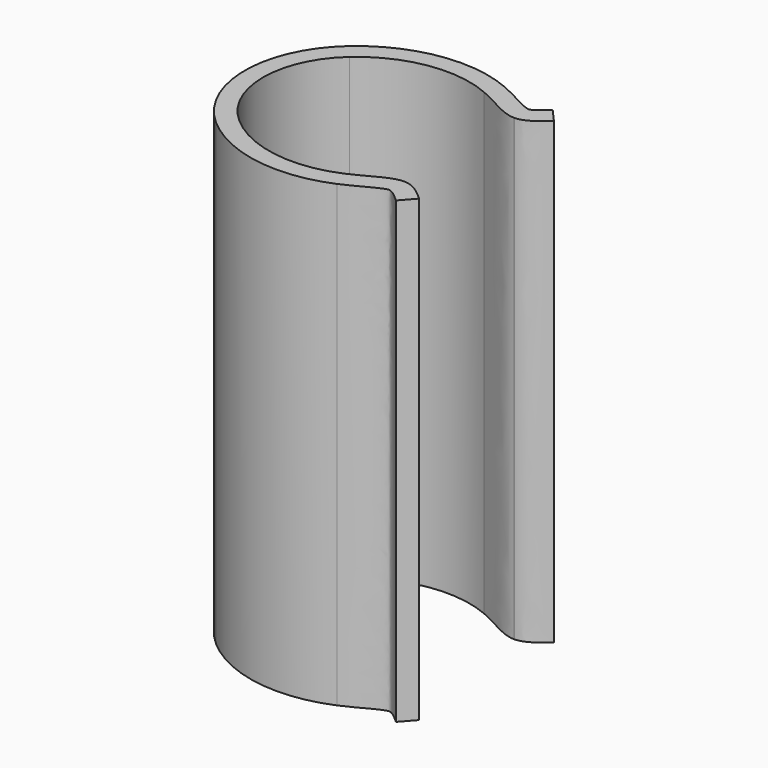
from build123d import *

# Parameters (mm, degrees)
F1_DEPTH = 50


# Not quite as in the source:
# - the dataset's text gives a spline's control points without its knots; the knots are read off the source's solid


with BuildPart() as f1:
    # F0 (on Top) → F1 (new body)
    with BuildSketch(Plane.XY):
        with BuildLine():
            ThreePointArc((13.0144933843, -2.085252316), (6.205255597, -2.9274153897), (0, 0))
            ThreePointArc((0, 0), (-3.3856217223, 7.5), (0, 15))
            ThreePointArc((0, 15), (6.205255597, 17.9274153897), (13.0144933843, 17.085252316))
            add(Edge.make_bspline(
                [(13.0144933843, 17.085252316), (14.9188937147, 16.2688716797), (16.5381459826, 15.0282447438), (17.9057964085, 15)],
                knots=[0, 0, 0, 0, 0.5457987429, 0.5457987429, 0.5457987429, 0.5457987429], degree=3))
            Line((17.9057964085, 15), (18, 15))
            add(Edge.make_bspline(
                [(18, 15), (19.0972191031, 15.0230880512), (20.0302273141, 15.8645970051), (20.9385249764, 16.6705846786)],
                knots=[0.5583835876, 0.5583835876, 0.5583835876, 0.5583835876, 1, 1, 1, 1], degree=3))
            Line((20.9385249764, 16.6705846786), (19.6110748236, 18.1665379172))
            add(Edge.make_bspline(
                [(13.8027239443, 18.9233743561), (14.3068240335, 18.7072663795), (15.238145762, 18.2426302327), (16.2240017083, 17.7036956521), (16.8916980315, 17.3645051566), (17.3205970551, 17.1709950677), (17.6036754274, 17.0697214684), (17.7738298239, 17.0243049098), (17.8699589675, 17.0058001031), (17.9347425496, 16.9993397818), (17.9615712094, 16.9993392849), (17.983336855, 17.0011188424), (18.031156036, 17.0095932598), (18.1317450508, 17.0407501327), (18.3942332342, 17.1702266018), (18.8744768256, 17.5122343093), (19.3516165065, 17.9363047964), (19.6110748236, 18.1665379172)],
                knots=[1.83025e-05, 1.83025e-05, 1.83025e-05, 1.83025e-05, 0.125, 0.25, 0.3125, 0.375, 0.4375, 0.46875, 0.5, 0.53125, 0.5625, 0.59375, 0.625, 0.6875, 0.75, 0.875, 1, 1, 1, 1], degree=3))
            ThreePointArc((13.8027239307, 18.9233743619), (5.8889598851, 19.9022462774), (-1.3228756555, 16.5))
            ThreePointArc((-1.3228756555, 16.5), (-5.3856217223, 7.5), (-1.3228756555, -1.5))
            ThreePointArc((-1.3228756555, -1.5), (5.8889598851, -4.9022462774), (13.8027239307, -3.9233743619))
            add(Edge.make_bspline(
                [(13.8027239443, -3.9233743561), (14.3068240335, -3.7072663795), (15.238145762, -3.2426302327), (16.2240017083, -2.7036956521), (16.8916980315, -2.3645051566), (17.3205970551, -2.1709950677), (17.6036754274, -2.0697214684), (17.7738298239, -2.0243049098), (17.8699589675, -2.0058001031), (17.9347425496, -1.9993397818), (17.9615712094, -1.9993392849), (17.983336855, -2.0011188424), (18.031156036, -2.0095932598), (18.1317450508, -2.0407501327), (18.3942332342, -2.1702266018), (18.8744768256, -2.5122343093), (19.3516165065, -2.9363047964), (19.6110748236, -3.1665379172)],
                knots=[1.83025e-05, 1.83025e-05, 1.83025e-05, 1.83025e-05, 0.125, 0.25, 0.3125, 0.375, 0.4375, 0.46875, 0.5, 0.53125, 0.5625, 0.59375, 0.625, 0.6875, 0.75, 0.875, 1, 1, 1, 1], degree=3))
            Line((19.6110748236, -3.1665379172), (20.9385249764, -1.6705846786))
            add(Edge.make_bspline(
                [(18, 0), (19.0972191031, -0.0230880512), (20.0302273141, -0.8645970051), (20.9385249764, -1.6705846786)],
                knots=[0.5583835876, 0.5583835876, 0.5583835876, 0.5583835876, 1, 1, 1, 1], degree=3))
            Line((18, 0), (17.9057964085, 0))
            add(Edge.make_bspline(
                [(13.0144933843, -2.085252316), (14.9188937147, -1.2688716797), (16.5381459826, -0.0282447438), (17.9057964085, 0)],
                knots=[0, 0, 0, 0, 0.5457987429, 0.5457987429, 0.5457987429, 0.5457987429], degree=3))
        make_face()
    extrude(amount=F1_DEPTH)


solid = f1.part
